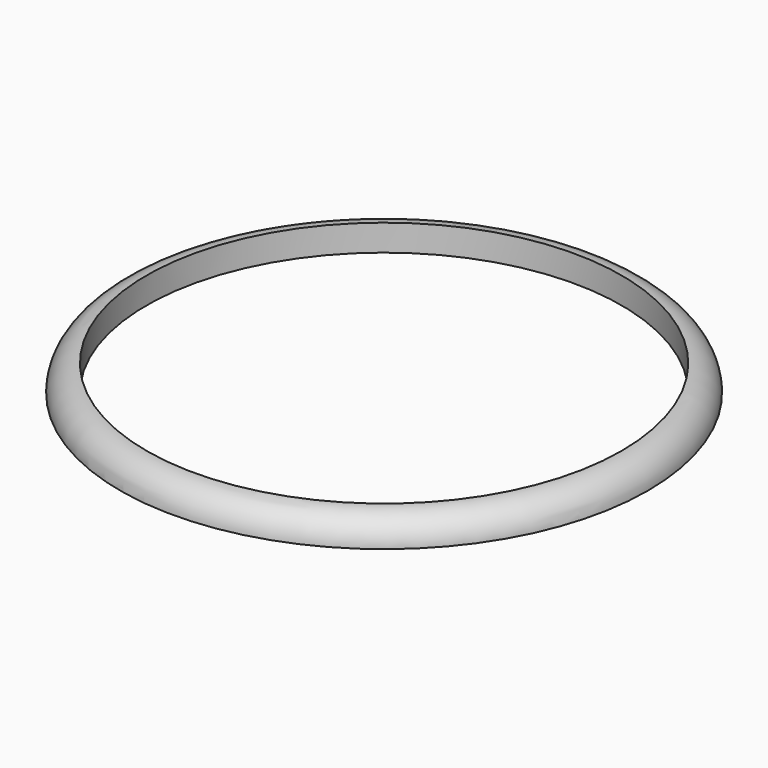
from build123d import *

# Parameters (mm, degrees)
F0_R     = 12.7
F0_R_2   = 11.43
F1_DEPTH = 1.27
F2_R     = 1.26999


# Not quite as in the source:
# - a fillet or chamfer is up to 0.001 mm smaller than in the source, because OpenCascade refuses the exact size


with BuildPart() as f1:
    # F0 (on Top) → F1 (new body)
    with BuildSketch(Plane.XY):
        Circle(F0_R)
        Circle(F0_R_2, mode=Mode.SUBTRACT)
    extrude(amount=F1_DEPTH)

    # F2 (radius 1.27 in the source; OpenCascade refuses exactly that, so slightly less here)
    f2_edges = [f1.edges().sort_by_distance(p)[0] for p in [
        (-12.7, 0, 1.27),
    ]]
    fillet(f2_edges, radius=F2_R)


solid = f1.part
